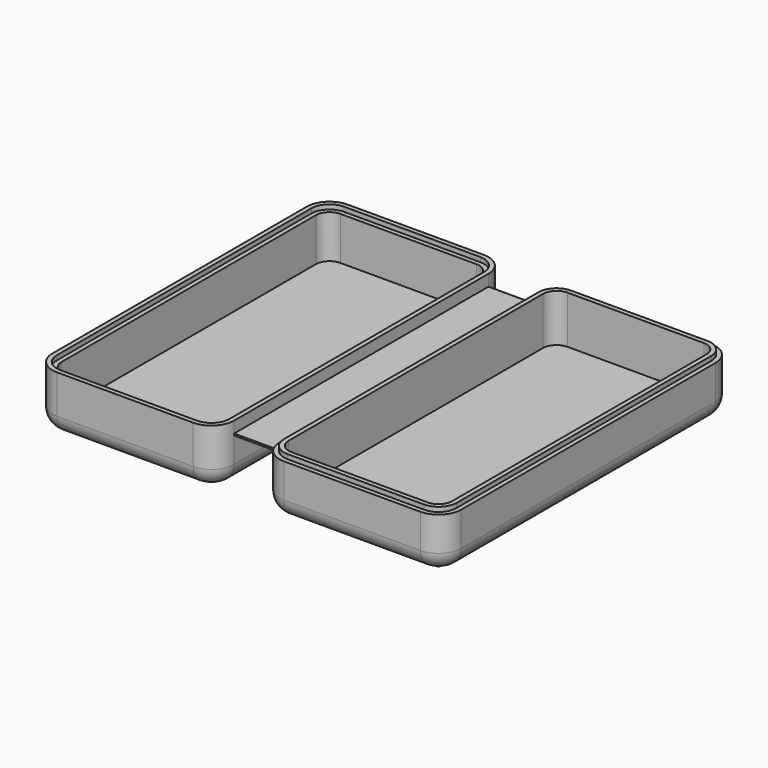
from build123d import *

# Parameters (mm, degrees)
F1_DEPTH      = 3.175
F1_DEPTH_BACK = 12.7
F0_W          = 12.7
F0_H          = 88.9
F2_DEPTH      = 0.508
F3_T          = 2.54
F3_T3_DEPTH   = 5.588
F3_T5_DEPTH   = 93.98
F5_DEPTH      = 1.27
F7_DEPTH      = 1.27
F8_ANGLE      = 90
F9_R          = 5.08
F10_W         = 38.1
F10_H         = 88.9
F11_DEPTH     = 0.762
F12_W         = 38.1
F12_H         = 88.9
F12_TEXT_SIZE = 41.237950279
F13_DEPTH     = 0.508


# Not quite as in the source:
# - a shell that OpenCascade refuses in one call is made with other operations: the cavity is built on its own and cut out
# - Text() gives the source's letters only with a copy of the font that has no kerning and outlines rounded to 1/6400 em; it was checked with that copy


with BuildPart() as f1:
    # F0 (on Top) → F1 (new body, two sides)
    with BuildSketch(Plane.XY) as f1_sk:
        with BuildLine():
            Line((-6.35, -44.45), (-6.35, 44.45))
            ThreePointArc((-6.35, 44.45), (-8.2098719395, 48.9401280605), (-12.7, 50.8))
            Line((-12.7, 50.8), (-50.8, 50.8))
            ThreePointArc((-50.8, 50.8), (-55.2901280605, 48.9401280605), (-57.15, 44.45))
            Line((-57.15, 44.45), (-57.15, 7.6511725783))
            Line((-57.15, 7.6511725783), (-57.15, -7.6511725783))
            Line((-57.15, -7.6511725783), (-57.15, -44.45))
            ThreePointArc((-57.15, -44.45), (-55.2901280605, -48.9401280605), (-50.8, -50.8))
            Line((-50.8, -50.8), (-12.7, -50.8))
            ThreePointArc((-12.7, -50.8), (-8.2098719395, -48.9401280605), (-6.35, -44.45))
        make_face()
    extrude(amount=F1_DEPTH)
    extrude(f1_sk.sketch, amount=-F1_DEPTH_BACK)



with BuildPart() as f1b:
    # F0 (on Top) → F1, piece 2 (new body, two sides)
    with BuildSketch(Plane.XY) as f1_2_sk:
        with BuildLine():
            ThreePointArc((57.15, 44.45), (55.2901280605, 48.9401280605), (50.8, 50.8))
            Line((50.8, 50.8), (12.7, 50.8))
            ThreePointArc((12.7, 50.8), (8.2098719395, 48.9401280605), (6.35, 44.45))
            Line((6.35, 44.45), (6.35, -44.45))
            ThreePointArc((6.35, -44.45), (8.2098719395, -48.9401280605), (12.7, -50.8))
            Line((12.7, -50.8), (50.8, -50.8))
            ThreePointArc((50.8, -50.8), (55.2901280605, -48.9401280605), (57.15, -44.45))
            Line((57.15, -44.45), (57.15, 44.45))
        make_face()
    extrude(amount=F1_DEPTH)
    extrude(f1_2_sk.sketch, amount=-F1_DEPTH_BACK)


with BuildPart() as f1_1:
    add(f1.part)

    add(f1b.part)  # F2 merges F1b
    # F0 (on Top) → F2 (join)
    with BuildSketch(Plane.XY):
        Rectangle(F0_W, F0_H)
    extrude(amount=-F2_DEPTH)

    # F3: shell of thickness 2.54, made by hand


with BuildPart() as f3_core1:
    # F3_t2: copy of F1
    add(f1_1.part)

    # the walls: a layer under each face that stays
    f3_faces = [f3_core1.faces().sort_by_distance(p)[0] for p in [
        (55.2901280605, 48.9401280605, -4.7625),
        (57.15, 0, -4.7625),
        (31.75, 50.8, -4.7625),
        (31.75, 0, -12.7),
        (55.2901280605, -48.9401280605, -4.7625),
        (8.2098719395, 48.9401280605, -4.7625),
        (6.35, 0, 1.5875),
        (8.2098719395, -48.9401280605, -4.7625),
        (31.75, -50.8, -4.7625),
        (6.35, 0, -6.604),
        (0, 44.45, -0.254),
        (0, 0, 0),
        (0, -44.45, -0.254),
        (0, 0, -0.508),
        (-8.2098719395, 48.9401280605, -4.7625),
        (-6.35, 0, 1.5875),
        (-8.2098719395, -48.9401280605, -4.7625),
        (-6.35, 0, -6.604),
        (-31.75, 50.8, -4.7625),
        (-31.75, 0, -12.7),
        (-31.75, -50.8, -4.7625),
        (-55.2901280605, 48.9401280605, -4.7625),
        (-57.15, 0, -4.7625),
        (-55.2901280605, -48.9401280605, -4.7625),
    ]]
    thicken(f3_faces, amount=-F3_T, mode=Mode.SUBTRACT)

    # F3_s4 → F3_t3 (cut)
    with BuildSketch(Plane.XY.offset(-3.048)):
        Polygon((6.3246, 44.4754), (8.89, 44.45), (8.89, 41.91), (6.35, 41.91), align=None)
        Polygon((6.3246, -44.4754), (8.89, -44.45), (8.89, -41.91), (6.35, -41.91), align=None)
        Polygon((-6.3246, 44.4754), (-6.35, 41.91), (-8.89, 41.91), (-8.89, 44.45), align=None)
        Polygon((-6.3246, -44.4754), (-6.35, -41.91), (-8.89, -41.91), (-8.89, -44.45), align=None)
    extrude(amount=F3_T3_DEPTH, mode=Mode.SUBTRACT)

    # F3_s6 → F3_t5 (cut)
    with BuildSketch(Plane.XZ.offset(-46.99)):
        Polygon((6.3246, 0.0254), (8.89, 0), (8.89, -2.54), (6.35, -2.54), align=None)
        Polygon((6.3246, -0.5334), (8.89, -0.508), (8.89, 2.032), (6.35, 2.032), align=None)
        Polygon((-6.3246, 0.0254), (-6.35, -2.54), (-8.89, -2.54), (-8.89, 0), align=None)
        Polygon((-6.3246, -0.5334), (-6.35, 2.032), (-8.89, 2.032), (-8.89, -0.508), align=None)
    extrude(amount=F3_T5_DEPTH, mode=Mode.SUBTRACT)


with BuildPart() as f1_2:
    add(f1_1.part)

    # what is left inside the walls is the cavity
    f3_cavity = [f3_core1.part.solids().sort_by_distance(p)[0] for p in [
        (31.75, -16.086667, 3.1496),
        (-31.75, -16.086667, -10.1346),
    ]]
    add(f3_cavity, mode=Mode.SUBTRACT)

    # F4 (on face) → F5 (cut)
    with BuildSketch(Plane.XY.offset(3.175)):
        with BuildLine():
            ThreePointArc((-7.62, 44.45), (-9.1078975516, 48.0421024484), (-12.7, 49.53))
            Line((-12.7, 49.53), (-50.8, 49.53))
            ThreePointArc((-50.8, 49.53), (-54.3921024484, 48.0421024484), (-55.88, 44.45))
            Line((-55.88, 44.45), (-55.88, -44.45))
            ThreePointArc((-55.88, -44.45), (-54.3921024484, -48.0421024484), (-50.8, -49.53))
            Line((-50.8, -49.53), (-12.7, -49.53))
            ThreePointArc((-12.7, -49.53), (-9.1078975516, -48.0421024484), (-7.62, -44.45))
            Line((-7.62, -44.45), (-7.62, 44.45))
        make_face()
        with BuildLine():
            ThreePointArc((-12.7, 48.26), (-10.0059231637, 47.1440768363), (-8.89, 44.45))
            Line((-8.89, 44.45), (-8.89, -44.45))
            ThreePointArc((-8.89, -44.45), (-10.0059231637, -47.1440768363), (-12.7, -48.26))
            Line((-12.7, -48.26), (-50.8, -48.26))
            ThreePointArc((-50.8, -48.26), (-53.4940768363, -47.1440768363), (-54.61, -44.45))
            Line((-54.61, -44.45), (-54.61, 44.45))
            ThreePointArc((-54.61, 44.45), (-53.4940768363, 47.1440768363), (-50.8, 48.26))
            Line((-50.8, 48.26), (-12.7, 48.26))
        make_face(mode=Mode.SUBTRACT)
    extrude(amount=-F5_DEPTH, mode=Mode.SUBTRACT)

    # F6 (on face) → F7 (cut)
    with BuildSketch(Plane.XY.offset(3.175)):
        with BuildLine():
            Line((57.15, -44.45), (57.15, 44.45))
            ThreePointArc((57.15, 44.45), (55.2901280605, 48.9401280605), (50.8, 50.8))
            Line((50.8, 50.8), (12.7, 50.8))
            ThreePointArc((12.7, 50.8), (8.2098719395, 48.9401280605), (6.35, 44.45))
            Line((6.35, 44.45), (6.35, -44.45))
            ThreePointArc((6.35, -44.45), (8.2098719395, -48.9401280605), (12.7, -50.8))
            Line((12.7, -50.8), (50.8, -50.8))
            ThreePointArc((50.8, -50.8), (55.2901280605, -48.9401280605), (57.15, -44.45))
        make_face()
        with BuildLine():
            ThreePointArc((55.88, -44.45), (54.3921024484, -48.0421024484), (50.8, -49.53))
            Line((50.8, -49.53), (12.7, -49.53))
            ThreePointArc((12.7, -49.53), (9.1078975516, -48.0421024484), (7.62, -44.45))
            Line((7.62, -44.45), (7.62, 44.45))
            ThreePointArc((7.62, 44.45), (9.1078975516, 48.0421024484), (12.7, 49.53))
            Line((12.7, 49.53), (50.8, 49.53))
            ThreePointArc((50.8, 49.53), (54.3921024484, 48.0421024484), (55.88, 44.45))
            Line((55.88, 44.45), (55.88, -44.45))
        make_face(mode=Mode.SUBTRACT)
    extrude(amount=-F7_DEPTH, mode=Mode.SUBTRACT)

    # F0 (on Top) → F8 (revolve)
    with BuildSketch(Plane.XY):
        with BuildLine():
            Line((-57.15, -7.6511725783), (-57.15, 7.6511725783))
            ThreePointArc((-57.15, 7.6511725783), (-60.3877414344, 0), (-57.15, -7.6511725783))
        make_face()
    revolve(axis=Axis((-57.15, 0, 0), (0, -1, 0)), revolution_arc=F8_ANGLE)

    # F9
    f9_edges = [f1_2.edges().sort_by_distance(p)[0] for p in [
        (55.290128, 48.940128, -12.7),
        (31.75, 50.8, -12.7),
        (8.209872, 48.940128, -12.7),
        (6.35, 0, -12.7),
        (8.209872, -48.940128, -12.7),
        (31.75, -50.8, -12.7),
        (55.290128, -48.940128, -12.7),
        (57.15, 0, -12.7),
        (-6.35, 0, -12.7),
        (-8.209872, 48.940128, -12.7),
        (-31.75, 50.8, -12.7),
        (-55.290128, 48.940128, -12.7),
        (-57.15, 0, -12.7),
        (-55.290128, -48.940128, -12.7),
        (-31.75, -50.8, -12.7),
        (-8.209872, -48.940128, -12.7),
    ]]
    fillet(f9_edges, radius=F9_R)

    # F10 (on face) → F11 (join)
    with BuildSketch(Plane(origin=(0, 0, -12.7), x_dir=(1, 0, 0), z_dir=(0, 0, -1))):
        with BuildLine():
            Line((12.7, -45.72), (50.8, -45.72))
            ThreePointArc((50.8, -45.72), (51.6980256121, -45.3480256121), (52.07, -44.45))
            Line((52.07, -44.45), (52.07, 44.45))
            ThreePointArc((52.07, 44.45), (51.6980256121, 45.3480256121), (50.8, 45.72))
            Line((50.8, 45.72), (12.7, 45.72))
            ThreePointArc((12.7, 45.72), (11.8019743879, 45.3480256121), (11.43, 44.45))
            Line((11.43, 44.45), (11.43, -44.45))
            ThreePointArc((11.43, -44.45), (11.8019743879, -45.3480256121), (12.7, -45.72))
        make_face()
        with Locations((31.75, 0)):
            Rectangle(F10_W, F10_H, mode=Mode.SUBTRACT)
    extrude(amount=F11_DEPTH)

    # F12 (on face) → F13 (join)
    with BuildSketch(Plane(origin=(0, 0, -12.7), x_dir=(1, 0, 0), z_dir=(0, 0, -1))):
        with BuildLine():
            ThreePointArc((-12.7, -45.72), (-11.8019743879, -45.3480256121), (-11.43, -44.45))
            Line((-11.43, -44.45), (-11.43, 44.45))
            ThreePointArc((-11.43, 44.45), (-11.8019743879, 45.3480256121), (-12.7, 45.72))
            Line((-12.7, 45.72), (-50.8, 45.72))
            ThreePointArc((-50.8, 45.72), (-51.6980256121, 45.3480256121), (-52.07, 44.45))
            Line((-52.07, 44.45), (-52.07, -44.45))
            ThreePointArc((-52.07, -44.45), (-51.6980256121, -45.3480256121), (-50.8, -45.72))
            Line((-50.8, -45.72), (-12.7, -45.72))
        make_face()
        with Locations((-31.75, 0)):
            Rectangle(F12_W, F12_H, mode=Mode.SUBTRACT)
        with Locations(Location((-45.72, 44.45), (0, 0, -90))):
            Text('BOX', F12_TEXT_SIZE, font='Tinos', text_align=(TextAlign.LEFT, TextAlign.BOTTOM))
    extrude(amount=F13_DEPTH)


solid = f1_2.part
